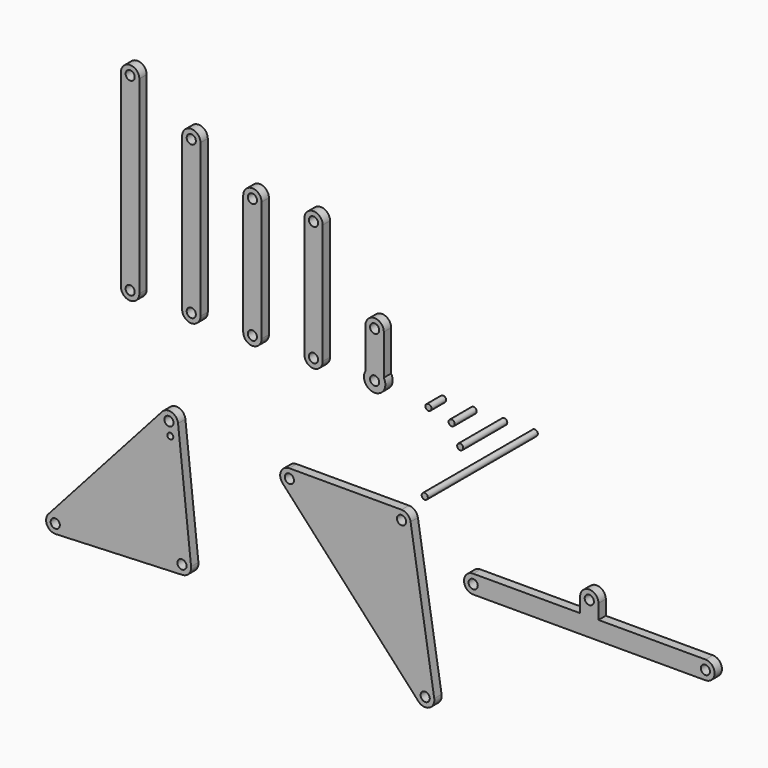
from build123d import *

# Parameters (mm, degrees)
F0_R     = 1.5
F2_DEPTH = 3
F0_R_2   = 0.9759621608
F3_R     = 1
F4_DEPTH = 6
F5_DEPTH = 9
F6_DEPTH = 18
F7_DEPTH = 45


# Not quite as in the source:
# - a feature names something its author has since deleted; it is built from what else it names


with BuildPart() as f2:
    # F0 (on Front) → F2 (new body)
    with BuildSketch(Plane.XZ):
        with BuildLine():
            Line((-93, 61.9), (-93, 0))
            ThreePointArc((-93, 0), (-90, -3), (-87, 0))
            Line((-87, 0), (-87, 61.9))
            ThreePointArc((-87, 61.9), (-90, 64.9), (-93, 61.9))
        make_face()
        with Locations((-90, 0)):
            Circle(F0_R, mode=Mode.SUBTRACT)
        with Locations((-90, 61.9)):
            Circle(F0_R, mode=Mode.SUBTRACT)
    extrude(amount=F2_DEPTH)


with BuildPart() as f2b:
    # F0 (on Front) → F2, piece 2 (new body)
    with BuildSketch(Plane.XZ):
        with BuildLine():
            Line((-73, 50), (-73, 0))
            ThreePointArc((-73, 0), (-70, -3), (-67, 0))
            Line((-67, 0), (-67, 50))
            ThreePointArc((-67, 50), (-70, 53), (-73, 50))
        make_face()
        with Locations((-70, 0)):
            Circle(F0_R, mode=Mode.SUBTRACT)
        with Locations((-70, 50)):
            Circle(F0_R, mode=Mode.SUBTRACT)
    extrude(amount=F2_DEPTH)


with BuildPart() as f2c:
    # F0 (on Front) → F2, piece 3 (new body)
    with BuildSketch(Plane.XZ):
        with BuildLine():
            Line((-53, 39.4), (-53, 0))
            ThreePointArc((-53, 0), (-50, -3), (-47, 0))
            Line((-47, 0), (-47, 39.4))
            ThreePointArc((-47, 39.4), (-50, 42.4), (-53, 39.4))
        make_face()
        with Locations((-50, 0)):
            Circle(F0_R, mode=Mode.SUBTRACT)
        with Locations((-50, 39.4)):
            Circle(F0_R, mode=Mode.SUBTRACT)
    extrude(amount=F2_DEPTH)


with BuildPart() as f2d:
    # F0 (on Front) → F2, piece 4 (new body)
    with BuildSketch(Plane.XZ):
        with BuildLine():
            Line((-33, 39.3), (-33, 0))
            ThreePointArc((-33, 0), (-30, -3), (-27, 0))
            Line((-27, 0), (-27, 39.3))
            ThreePointArc((-27, 39.3), (-30, 42.3), (-33, 39.3))
        make_face()
        with Locations((-30, 0)):
            Circle(F0_R, mode=Mode.SUBTRACT)
        with Locations((-30, 39.3)):
            Circle(F0_R, mode=Mode.SUBTRACT)
    extrude(amount=F2_DEPTH)


with BuildPart() as f2e:
    # F0 (on Front) → F2, piece 5 (new body)
    with BuildSketch(Plane.XZ):
        with BuildLine():
            Line((-70.0693181039, -73.1313235704), (-74.3264076657, -33.2579340924))
            ThreePointArc((-74.3264076657, -33.2579340924), (-76.3892099419, -30.7210473968), (-79.545154834, -31.576008902))
            Line((-79.545154834, -31.576008902), (-116.7527937374, -73.1600395777))
            ThreePointArc((-116.7527937374, -73.1600395777), (-117.2299941009, -76.4411409069), (-114.393432354, -78.1579005219))
            Line((-114.393432354, -78.1579005219), (-72.9287038888, -76.4472593243))
            ThreePointArc((-72.9287038888, -76.4472593243), (-70.7804128493, -75.4089504152), (-70.0693181039, -73.1313235704))
        make_face()
        with Locations((-114.5170931635, -75.1604502714)):
            Circle(F0_R, mode=Mode.SUBTRACT)
        with Locations((-73.0523646983, -73.4498090738)):
            Circle(F0_R, mode=Mode.SUBTRACT)
        with Locations((-76.8650740152, -37.7386403628)):
            Circle(F0_R_2, mode=Mode.SUBTRACT)
        with Locations((-77.30945426, -33.5764195958)):
            Circle(F0_R, mode=Mode.SUBTRACT)
    extrude(amount=F2_DEPTH)


with BuildPart() as f2f:
    # F0 (on Front) → F2, piece 6 (new body)
    with BuildSketch(Plane.XZ):
        with BuildLine():
            Line((-1.2049454206, -34.3364864443), (-37.9049454206, -34.3364864443))
            ThreePointArc((-37.9049454206, -34.3364864443), (-40.6516320173, -36.1299572323), (-40.1142504973, -39.3660112847))
            Line((-40.1142504973, -39.3660112847), (4.3323435081, -87.7497924651))
            ThreePointArc((4.3323435081, -87.7497924651), (7.8489363001, -88.4204525868), (9.503920902, -85.2459863591))
            Line((9.503920902, -85.2459863591), (1.7573268966, -36.8622051786))
            ThreePointArc((1.7573268966, -36.8622051786), (0.7414815885, -35.0536325509), (-1.2049454206, -34.3364864443))
        make_face()
        with Locations((-37.9049454206, -37.3364864443)):
            Circle(F0_R, mode=Mode.SUBTRACT)
        with Locations((6.5416485849, -85.7202676247)):
            Circle(F0_R, mode=Mode.SUBTRACT)
        with Locations((-1.2049454206, -37.3364864443)):
            Circle(F0_R, mode=Mode.SUBTRACT)
    extrude(amount=F2_DEPTH)


with BuildPart() as f2g:
    # F0 (on Front) → F2, piece 7 (new body)
    with BuildSketch(Plane.XZ):
        with BuildLine():
            Line((57.2455593391, -45.1364864443), (22.2455593391, -45.1364864443))
            ThreePointArc((22.2455593391, -45.1364864443), (19.2455593391, -48.1364864443), (22.2455593391, -51.1364864443))
            Line((22.2455593391, -51.1364864443), (98.2455593391, -51.1364864443))
            ThreePointArc((98.2455593391, -51.1364864443), (101.2455593391, -48.1364864443), (98.2455593391, -45.1364864443))
            Line((98.2455593391, -45.1364864443), (63.2455593391, -45.1364864443))
            Line((63.2455593391, -45.1364864443), (63.2455593391, -40.3364864443))
            ThreePointArc((63.2455593391, -40.3364864443), (60.2455593391, -37.3364864443), (57.2455593391, -40.3364864443))
            Line((57.2455593391, -40.3364864443), (57.2455593391, -45.1364864443))
        make_face()
        with Locations((22.2455593391, -48.1364864443)):
            Circle(F0_R, mode=Mode.SUBTRACT)
        with Locations((60.2455593391, -40.3364864443)):
            Circle(F0_R, mode=Mode.SUBTRACT)
        with Locations((98.2455593391, -48.1364864443)):
            Circle(F0_R, mode=Mode.SUBTRACT)
    extrude(amount=F2_DEPTH)


with BuildPart() as f2h:
    # F0 (on Front) → F2, piece 8 (new body)
    with BuildSketch(Plane.XZ):
        with BuildLine():
            Line((-7, 1.8027756377), (-7, 15))
            ThreePointArc((-7, 15), (-10, 18), (-13, 15))
            Line((-13, 15), (-13, 1.8027756377))
            ThreePointArc((-13, 1.8027756377), (-10, -3.5), (-7, 1.8027756377))
        make_face()
        with Locations((-10, 0)):
            Circle(F0_R, mode=Mode.SUBTRACT)
        with Locations((-10, 15)):
            Circle(F0_R, mode=Mode.SUBTRACT)
    extrude(amount=F2_DEPTH)


with BuildPart() as f4:
    # F3 (on Front) → F4 (new body)
    with BuildSketch(Plane.XZ):
        with Locations((10, 0)):
            Circle(F3_R)
    extrude(amount=F4_DEPTH)


with BuildPart() as f5:
    # F3 (on Front) → F5 (new body)
    with BuildSketch(Plane.XZ):
        with Locations((20, 0)):
            Circle(F3_R)
    extrude(amount=F5_DEPTH)


with BuildPart() as f6:
    # F3 (on Front) → F6 (new body)
    with BuildSketch(Plane.XZ):
        with Locations((30, 0)):
            Circle(F3_R)
    extrude(amount=F6_DEPTH)


with BuildPart() as f7:
    # F3 (on Front) → F7 (new body)
    with BuildSketch(Plane.XZ):
        with Locations((40, 0)):
            Circle(F3_R)
    extrude(amount=F7_DEPTH)


solid = Compound([f2.part, f2b.part, f2c.part, f2d.part, f2e.part, f2f.part, f2g.part, f2h.part, f4.part, f5.part, f6.part, f7.part])
